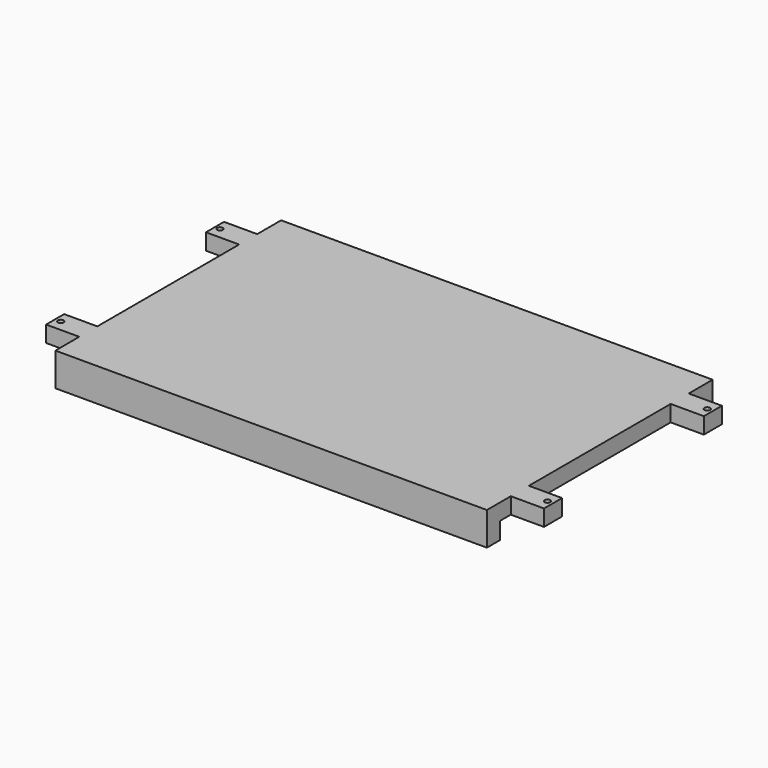
from build123d import *

# Parameters (mm, degrees)
F1_DEPTH = 4.9
F2_R     = 0.85
F3_DEPTH = 4.901
F4_W     = 130
F4_H     = 4
F5_DEPTH = 4.9
F6_W     = 130
F6_H     = 5
F7_DEPTH = 10


with BuildPart() as f1:
    # F0 (on Top) → F1 (new body)
    with BuildSketch(Plane.XY):
        Polygon((-75, -33.5), (75, -33.5), (75, -26.7), (65, -26.7), (65, 26.7), (75, 26.7), (75, 33.5), (-75, 33.5), (-75, 26.7), (-65, 26.7), (-65, -26.7), (-75, -26.7), align=None)
    extrude(amount=F1_DEPTH)

    # F2 (on face) → F3 (cut, through all)
    with BuildSketch(Plane.XY.offset(4.9)):
        with Locations((-73.5, 30.1)):
            Circle(F2_R)
        with Locations((-73.3, -30.1)):
            Circle(F2_R)
        with Locations((73.3, 30.1)):
            Circle(F2_R)
        with Locations((73.3, -30.1)):
            Circle(F2_R)
    extrude(amount=-F3_DEPTH, mode=Mode.SUBTRACT)

    # F4 (on face) → F5 (join)
    with BuildSketch(Plane.XY.offset(4.9)):
        with Locations((0, 35.5)):
            Rectangle(F4_W, F4_H)
        with Locations((0, -35.5)):
            Rectangle(F4_W, F4_H)
    extrude(amount=-F5_DEPTH)

    # F6 (on face) → F7 (join)
    with BuildSketch(Plane.XY.offset(4.9)):
        with Locations((0, 40)):
            Rectangle(F6_W, F6_H)
        with Locations((0, -40)):
            Rectangle(F6_W, F6_H)
    extrude(amount=-F7_DEPTH)


solid = f1.part
